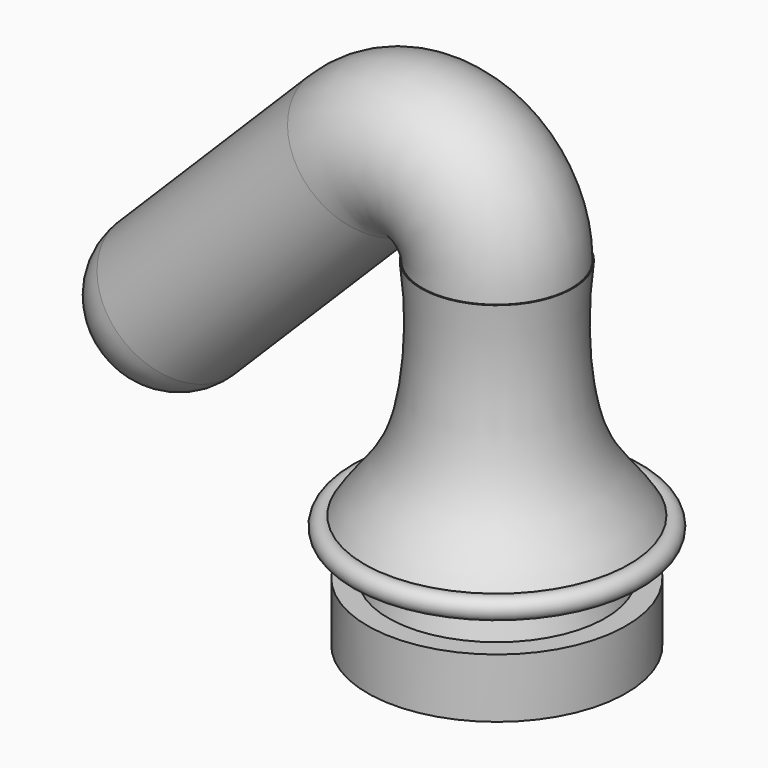
from build123d import *

# Parameters (mm, degrees)
F5_R     = 5.5475
F6_ANGLE = 135
F7_DEPTH = 25
F8_R     = 5


with BuildPart() as f1:
    # F0 (on Front) → F1 (revolve)
    with BuildSketch(Plane.XZ):
        with BuildLine():
            Line((0, -72.7080839413), (0, -54.644279182))
            Line((0, -54.644279182), (-5.6319482939, -54.644279182))
            add(Edge.make_bspline(
                [(-5.6319482939, -54.644279182), (-5.1288321088, -58.6179507974), (-5.6211565128, -66.4424929302), (-8.3574508563, -69.170647696), (-9.6287897185, -70.9672772938), (-9.8312023567, -71.3003521886)],
                knots=[0.5403591349, 0.5403591349, 0.5403591349, 0.5403591349, 0.6019546263, 0.6513447325, 0.6619692363, 0.6619692363, 0.6619692363, 0.6619692363], degree=3))
            add(Edge.make_bspline(
                [(-9.8312023567, -71.3003521886), (-10.0998646212, -71.7424424467), (-10.3286150665, -72.2109833189), (-10.4702698771, -72.7080839413)],
                knots=[0.6619692363, 0.6619692363, 0.6619692363, 0.6619692363, 0.6760711386, 0.6760711386, 0.6760711386, 0.6760711386], degree=3))
            Line((-10.4702698771, -72.7080839413), (0, -72.7080839413))
        make_face()
        with BuildLine():
            add(Edge.make_bspline(
                [(-9.8312023567, -71.3003521886), (-10.0998646212, -71.7424424467), (-10.3286150665, -72.2109833189), (-10.4702698771, -72.7080839413)],
                knots=[0.6619692363, 0.6619692363, 0.6619692363, 0.6619692363, 0.6760711386, 0.6760711386, 0.6760711386, 0.6760711386], degree=3))
            ThreePointArc((-9.8312023567, -71.3003521886), (-10.8545430206, -71.6847110766), (-10.4702698771, -72.7080839413))
        make_face()
    revolve(axis=Axis((0, 0, -15.5616570242), (0, 0, -1)))

    # F5 (on face) → F6 (revolve)
    with BuildSketch(Plane.XY.offset(-54.644279182)):
        Circle(F5_R)
    revolve(axis=Axis((-5.6319482939, 2.586, -54.644279182), (0, -1, 0)), revolution_arc=F6_ANGLE)

    # F7 (add): a face of the model
    f7_faces = [f1.faces().sort_by_distance(p)[0] for p in [
        (-9.6143371239, 0, -50.661890352),
    ]]
    extrude(f7_faces, amount=F7_DEPTH)

    # F8
    f8_edges = [f1.edges().sort_by_distance(p)[0] for p in [
        (-23.369332, 0, -72.262235),
    ]]
    fillet(f8_edges, radius=F8_R)


with BuildPart() as f4:
    # F3 (on Right) → F4 (revolve)
    with BuildSketch(Plane.YZ):
        Polygon((1.2, -51.5964031219), (0.894790981, -51.5964031219), (7.7754920349, -76.3285309076), (9.0201694891, -76.3285309076), (9.0201694891, -79.8001212753), (9.6011694891, -79.8001212753), (9.6011694891, -75.3971212753), (8.0541694891, -75.3971212753), align=None)
    revolve(axis=Axis((0, 0, -65.6982621986), (0, 0, 1)))


solid = Compound([f1.part, f4.part])
